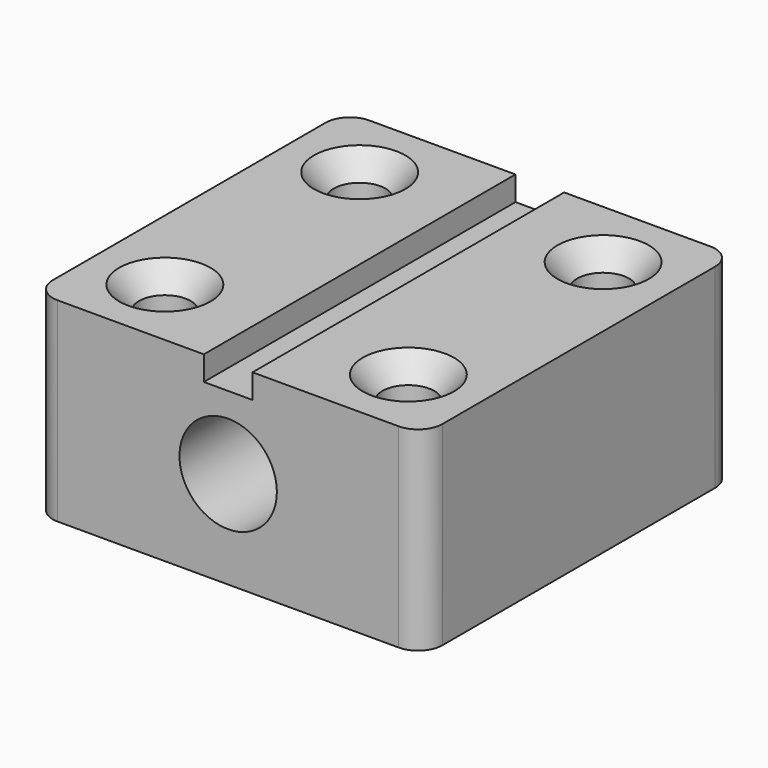
from build123d import *

# Parameters (mm, degrees)
F1_DEPTH       = 50.8
F3_D           = 13.49248
F3_CSINK_D     = 23.8252
F3_CSINK_ANGLE = 82
F4_R           = 6.35
F5_W           = 12.7
F5_H           = 101.6
F6_DEPTH       = 6.35
F7_R           = 12.7
F8_DEPTH       = 101.601


# Not quite as in the source:
# - a feature of the source that left no trace in its solid (it failed there, or was rolled back) is left out


with BuildPart() as f1:
    # F0 (on Front) → F1 (new body, symmetric)
    with BuildSketch(Plane.XZ):
        Polygon((12.601675614, 25.4), (-50.8, 25.4), (-50.8, -25.4), (50.8, -25.4), (50.8, 25.4), align=None)
    extrude(amount=F1_DEPTH, both=True)

    # F3 (through all)
    with Locations(Plane.XY.offset(25.4)):
        with Locations((-31.75, 31.75), (31.75, 31.75), (-31.75, -31.75), (31.75, -31.75)):
            CounterSinkHole(F3_D / 2, F3_CSINK_D / 2, counter_sink_angle=F3_CSINK_ANGLE)

    # F4
    f4_edges = [f1.edges().sort_by_distance(p)[0] for p in [
        (-50.8, 50.8, 0),
        (-50.8, -50.8, 0),
        (50.8, -50.8, 0),
        (50.8, 50.8, 0),
    ]]
    fillet(f4_edges, radius=F4_R)

    # F5 (on face) → F6 (cut)
    with BuildSketch(Plane.XY.offset(25.4)):
        Rectangle(F5_W, F5_H)
    extrude(amount=-F6_DEPTH, mode=Mode.SUBTRACT)

    # F7 (on face) → F8 (cut, through all)
    with BuildSketch(Plane.XZ.offset(50.8)):
        Circle(F7_R)
    extrude(amount=-F8_DEPTH, mode=Mode.SUBTRACT)


solid = f1.part
